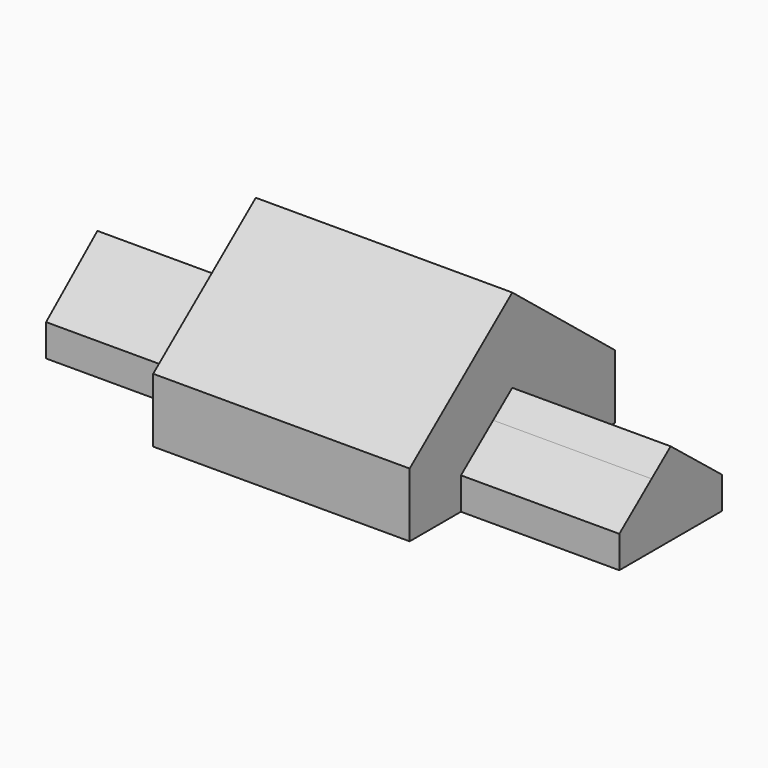
from build123d import *

# Parameters (mm, degrees)
F1_DEPTH = 10
F0_W     = 24.7
F0_H     = 20
F2_DEPTH = 5
F5_DEPTH = 24.7
F6_DEPTH = 40
F9_DEPTH = 24.7


with BuildPart() as f1:
    # F0 (on Top) → F1 (new body)
    with BuildSketch(Plane.XY):
        Polygon((-20, 25), (-20, 15), (-20, -5), (-20, -15), (20, -15), (20, -5), (20, 15), (20, 25), align=None)
    extrude(amount=F1_DEPTH)

    # F0 (on Top) → F2 (join)
    with BuildSketch(Plane.XY):
        with Locations((-32.35, 5)):
            Rectangle(F0_W, F0_H)
        Polygon((-20, 25), (-20, 15), (-20, -5), (-20, -15), (20, -15), (20, -5), (20, 15), (20, 25), align=None)
        with Locations((32.35, 5)):
            Rectangle(F0_W, F0_H)
    extrude(amount=F2_DEPTH)

    # F4 (on offset) → F5 (join)
    with BuildSketch(Plane.YZ.offset(20)):
        Polygon((-5, 5), (15, 5), (8.7127050693, 10), (1.2872949307, 10), align=None)
        Polygon((1.2872949307, 10), (8.7127050693, 10), (5, 12.9525456578), align=None)
    extrude(amount=F5_DEPTH)

    # F4 (on offset) → F6 (join)
    with BuildSketch(Plane.YZ.offset(20)):
        Polygon((5, 12.9525456578), (8.7127050693, 10), (25, 10), (5, 26.0377600789), (-15, 10), (1.2872949307, 10), align=None)
        Polygon((1.2872949307, 10), (8.7127050693, 10), (5, 12.9525456578), align=None)
    extrude(amount=-F6_DEPTH)

    # F8 (on offset) → F9 (join)
    with BuildSketch(Plane(origin=(-20, 0, 0), x_dir=(0, -1, 0), z_dir=(-1, 0, 0))):
        Polygon((-15, 5), (5, 5), (-5, 13.4582445025), align=None)
    extrude(amount=F9_DEPTH)


solid = f1.part
